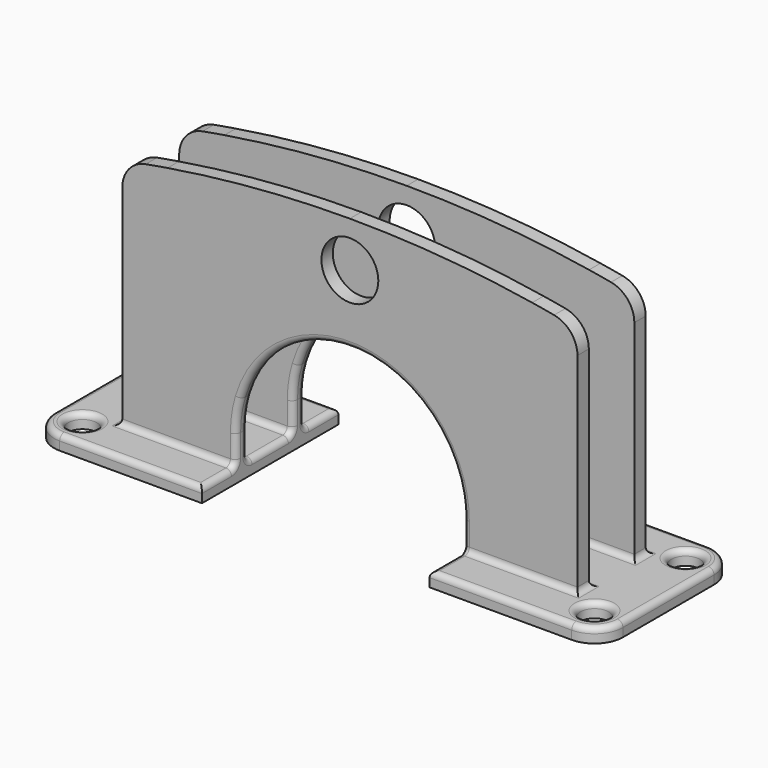
from build123d import *

# Parameters (mm, degrees)
F0_R     = 3.175
F1_DEPTH = 3.175
F2_W     = 50.8
F2_H     = 38.1
F3_DEPTH = 3.176
F4_R     = 6.35
F5_DEPTH = 38.1
F6_W     = 9.525
F6_H     = 46.7782413843
F6_H_2   = 54.8217586157
F6_W_2   = 12.7
F7_DEPTH = 114.301
F8_F1_R  = 1.27
F8_F2_R  = 1.27


with BuildPart() as f1:
    # F0 (on Top) → F1 (new body)
    with BuildSketch(Plane.XY):
        with BuildLine():
            Line((57.15, 19.05), (-57.15, 19.05))
            ThreePointArc((-57.15, 19.05), (-61.6401280605, 17.1901280605), (-63.5, 12.7))
            Line((-63.5, 12.7), (-63.5, -12.7))
            ThreePointArc((-63.5, -12.7), (-61.6401280605, -17.1901280605), (-57.15, -19.05))
            Line((-57.15, -19.05), (57.15, -19.05))
            ThreePointArc((57.15, -19.05), (61.6401280605, -17.1901280605), (63.5, -12.7))
            Line((63.5, -12.7), (63.5, 12.7))
            ThreePointArc((63.5, 12.7), (61.6401280605, 17.1901280605), (57.15, 19.05))
        make_face()
        with Locations((-57.15, -12.7)):
            Circle(F0_R, mode=Mode.SUBTRACT)
        with Locations((57.15, -12.7)):
            Circle(F0_R, mode=Mode.SUBTRACT)
        with Locations((-57.15, 12.7)):
            Circle(F0_R, mode=Mode.SUBTRACT)
        with Locations((57.15, 12.7)):
            Circle(F0_R, mode=Mode.SUBTRACT)
    extrude(amount=F1_DEPTH)

    # F2 (on face) → F3 (cut, through all)
    with BuildSketch(Plane.XY.offset(3.175)):
        Rectangle(F2_W, F2_H)
    extrude(amount=-F3_DEPTH, mode=Mode.SUBTRACT)

    # F4 (on face) → F5 (join, through all)
    with BuildSketch(Plane.XZ.offset(19.05)):
        with BuildLine():
            ThreePointArc((24.3291167869, 16.8225390625), (25.1308532126, 13.2128471777), (25.4, 9.525))
            Line((25.4, 9.525), (25.4, 3.175))
            Line((25.4, 3.175), (50.8, 3.175))
            Line((50.8, 3.175), (50.8, 49.9532413843))
            ThreePointArc((50.8, 49.9532413843), (49.3264675635, 54.0204964909), (45.5897435897, 56.2001193685))
            ThreePointArc((45.5897435897, 56.2001193685), (43.1458510734, 56.633680503), (40.6978385912, 57.0433398438))
            ThreePointArc((40.6978385912, 57.0433398437), (41.130456555, 53.6162560865), (41.275, 50.165))
            ThreePointArc((41.275, 50.165), (36.7954475471, 31.4641801033), (24.3291167869, 16.8225390625))
        make_face()
        with BuildLine():
            ThreePointArc((0, 60.325), (-20.414966075, 59.5032557017), (-40.6978385912, 57.0433398438))
            ThreePointArc((-40.6978385912, 57.0433398437), (-38.2302816535, 34.6063628588), (-24.3291167869, 16.8225390625))
            ThreePointArc((-24.3291167869, 16.8225390625), (0, 34.925), (24.3291167869, 16.8225390625))
            ThreePointArc((24.3291167869, 16.8225390625), (36.7954475471, 31.4641801033), (41.275, 50.165))
            ThreePointArc((41.275, 50.165), (41.130456555, 53.6162560865), (40.6978385912, 57.0433398437))
            ThreePointArc((40.6978385912, 57.0433398438), (20.414966075, 59.5032557017), (0, 60.325))
        make_face()
        with Locations((0, 50.165)):
            Circle(F4_R, mode=Mode.SUBTRACT)
        with BuildLine():
            Line((-50.8, 49.9532413843), (-50.8, 3.175))
            Line((-50.8, 3.175), (-25.4, 3.175))
            Line((-25.4, 3.175), (-25.4, 9.525))
            ThreePointArc((-25.4, 9.525), (-25.1308532126, 13.2128471777), (-24.3291167869, 16.8225390625))
            ThreePointArc((-24.3291167869, 16.8225390625), (-38.2302816535, 34.6063628588), (-40.6978385912, 57.0433398437))
            ThreePointArc((-40.6978385912, 57.0433398438), (-43.1458510734, 56.633680503), (-45.5897435897, 56.2001193685))
            ThreePointArc((-45.5897435897, 56.2001193685), (-49.3264675635, 54.0204964909), (-50.8, 49.9532413843))
        make_face()
    extrude(amount=-F5_DEPTH)

    # F6 (on face) → F7 (cut, through all)
    with BuildSketch(Plane.YZ.offset(50.8)):
        with Locations((-14.2875, 26.5641206921)):
            Rectangle(F6_W, F6_H)
        with Locations((-14.2875, 77.3641206921)):
            Rectangle(F6_W, F6_H_2)
        with Locations((14.2875, 26.5641206921)):
            Rectangle(F6_W, F6_H)
        with Locations((14.2875, 77.3641206921)):
            Rectangle(F6_W, F6_H_2)
        with Locations((0, 26.5641206921)):
            Rectangle(F6_W_2, F6_H)
        with Locations((0, 77.3641206921)):
            Rectangle(F6_W_2, F6_H_2)
    extrude(amount=-F7_DEPTH, mode=Mode.SUBTRACT)

    # F8: fillet of radius 1.27 on 32 edges, made by hand

    # F8_f1
    f8_f1_edges = [f1.edges().sort_by_distance(p)[0] for p in [
        (-38.1, 9.525, 3.175),
        (-50.8, 7.9375, 3.175),
        (-38.1, 6.35, 3.175),
        (-38.1, -6.35, 3.175),
        (-50.8, -7.9375, 3.175),
        (-38.1, -9.525, 3.175),
        (38.1, 9.525, 3.175),
        (38.1, -9.525, 3.175),
        (50.8, -7.9375, 3.175),
        (38.1, -6.35, 3.175),
        (38.1, 6.35, 3.175),
        (50.8, 7.9375, 3.175),
    ]]
    fillet(f8_f1_edges, radius=F8_F1_R)

    # F8_f2
    f8_f2_edges = [f1.edges().sort_by_distance(p)[0] for p in [
        (-41.275, -19.05, 3.175),
        (-61.6401280605, -17.1901280605, 3.175),
        (-63.5, 0, 3.175),
        (-61.6401280605, 17.1901280605, 3.175),
        (-41.275, 19.05, 3.175),
        (-25.4, 14.9225, 3.175),
        (-25.4, 0, 3.175),
        (-25.4, -14.9225, 3.175),
        (-60.325, -12.7, 3.175),
        (-60.325, 12.7, 3.175),
        (25.4, 14.9225, 3.175),
        (41.275, 19.05, 3.175),
        (61.6401280605, 17.1901280605, 3.175),
        (63.5, 0, 3.175),
        (61.6401280605, -17.1901280605, 3.175),
        (41.275, -19.05, 3.175),
        (25.4, -14.9225, 3.175),
        (25.4, 0, 3.175),
        (53.975, 12.7, 3.175),
        (53.975, -12.7, 3.175),
        (25.4, -5.9780256121, 3.5469743879),
        (25.4, 5.9780256121, 3.5469743879),
        (25.4, -9.8969743879, 3.5469743879),
        (25.4, 9.8969743879, 3.5469743879),
        (-25.4, -9.8969743879, 3.5469743879),
        (-25.4, -5.9780256121, 3.5469743879),
        (-25.4, 5.9780256121, 3.5469743879),
        (-25.4, 9.8969743879, 3.5469743879),
    ]]
    fillet(f8_f2_edges, radius=F8_F2_R)


solid = f1.part
